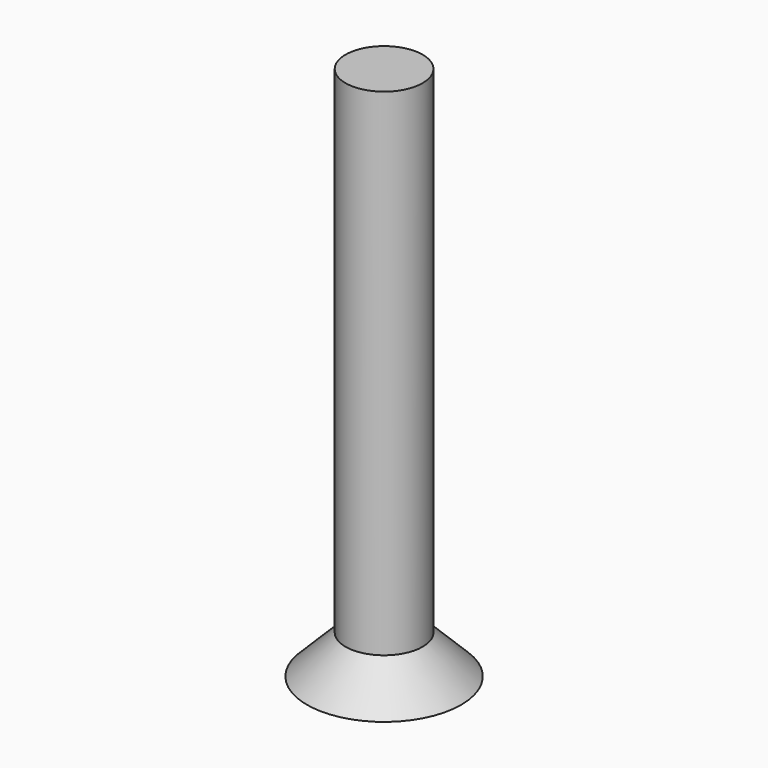
from build123d import *

# Parameters (mm, degrees)
F0_R     = 3
F1_DEPTH = 1.5
F2_SIZE  = 1.49999
F3_DEPTH = 19.3


# Not quite as in the source:
# - a fillet or chamfer is up to 0.001 mm smaller than in the source, because OpenCascade refuses the exact size


with BuildPart() as f1:
    # F0 (on Top) → F1 (new body)
    with BuildSketch(Plane.XY):
        Circle(F0_R)
    extrude(amount=F1_DEPTH)

    # F2 (size 1.5 in the source; OpenCascade refuses exactly that, so slightly less here)
    f2_edges = [f1.edges().sort_by_distance(p)[0] for p in [
        (-3, 0, 1.5),
    ]]
    chamfer(f2_edges, length=F2_SIZE)

    # F3 (add): a face of the model
    f3_faces = [f1.faces().sort_by_distance(p)[0] for p in [
        (0, 0, 1.5),
    ]]
    extrude(f3_faces, amount=F3_DEPTH)


solid = f1.part
